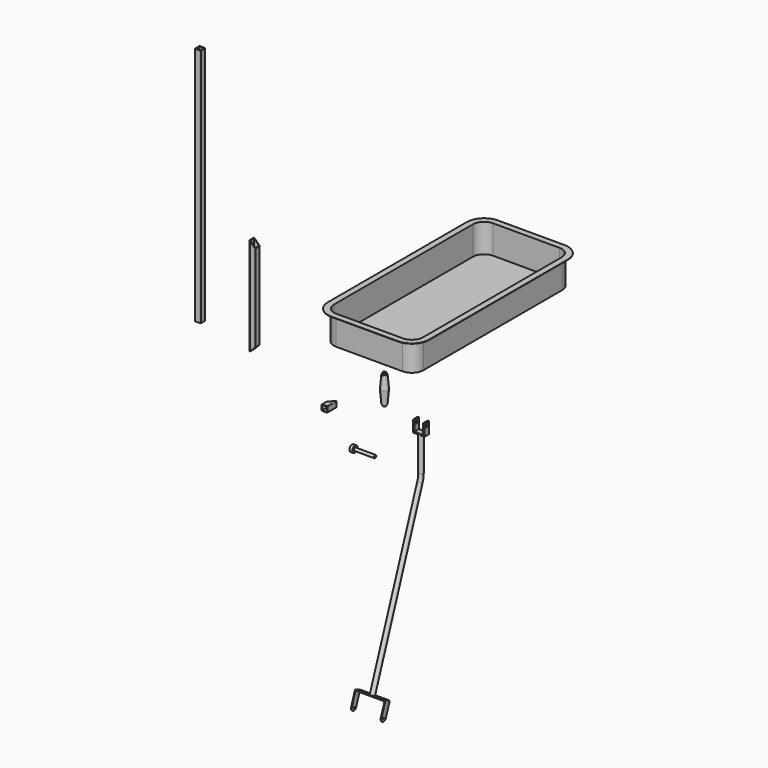
from build123d import *

# Parameters (mm, degrees)
F1_DEPTH  = 1054.1
F3_DEPTH  = 431.8
F5_DEPTH  = 50.8
F7_DEPTH  = 25.4
F9_DEPTH  = 25.4
F13_DEPTH = 127
F14_T     = -1.524
F16_DEPTH = 1.524
F18_DEPTH = 25.4
F19_R     = 9.525
F23_R     = 6.35
F24_DEPTH = 50.8
F25_W     = 127
F25_H     = 25.4
F25_R     = 9.525
F26_DEPTH = 3.175
F28_DEPTH = 25.4
F29_R     = 3.175
F30_DEPTH = 133.35
F31_R     = 12.69999


# Not quite as in the source:
# - a fillet or chamfer is up to 0.001 mm smaller than in the source, because OpenCascade refuses the exact size


with BuildPart() as f1:
    # F0 (on Top) → F1 (new body)
    with BuildSketch(Plane.XY):
        with BuildLine():
            ThreePointArc((-1008.6002467976, 278.8412709408), (-1007.9306928994, 277.224824839), (-1006.3142467976, 276.5552709408))
            Line((-1006.3142467976, 276.5552709408), (-985.4862467976, 276.5552709408))
            ThreePointArc((-985.4862467976, 276.5552709408), (-983.8698006958, 277.224824839), (-983.2002467976, 278.8412709408))
            Line((-983.2002467976, 278.8412709408), (-983.2002467976, 299.6692709408))
            ThreePointArc((-983.2002467976, 299.6692709408), (-983.8698006958, 301.2857170426), (-985.4862467976, 301.9552709408))
            Line((-985.4862467976, 301.9552709408), (-1006.3142467976, 301.9552709408))
            ThreePointArc((-1006.3142467976, 301.9552709408), (-1007.9306928994, 301.2857170426), (-1008.6002467976, 299.6692709408))
            Line((-1008.6002467976, 299.6692709408), (-1008.6002467976, 278.8412709408))
        make_face()
        with BuildLine():
            ThreePointArc((-1006.5682467976, 299.6692709408), (-1006.49385192, 299.8488760632), (-1006.3142467976, 299.9232709408))
            Line((-1006.3142467976, 299.9232709408), (-985.4862467976, 299.9232709408))
            ThreePointArc((-985.4862467976, 299.9232709408), (-985.3066416751, 299.8488760632), (-985.2322467976, 299.6692709408))
            Line((-985.2322467976, 299.6692709408), (-985.2322467976, 278.8412709408))
            ThreePointArc((-985.2322467976, 278.8412709408), (-985.3066416751, 278.6616658184), (-985.4862467976, 278.5872709408))
            Line((-985.4862467976, 278.5872709408), (-1006.3142467976, 278.5872709408))
            ThreePointArc((-1006.3142467976, 278.5872709408), (-1006.49385192, 278.6616658184), (-1006.5682467976, 278.8412709408))
            Line((-1006.5682467976, 278.8412709408), (-1006.5682467976, 299.6692709408))
        make_face(mode=Mode.SUBTRACT)
    extrude(amount=F1_DEPTH)


with BuildPart() as f3:
    # F2 (on Top) → F3 (new body)
    with BuildSketch(Plane.XY):
        with BuildLine():
            ThreePointArc((-720.8398963928, 218.5947193251), (-720.1703424946, 216.9782732233), (-718.5538963928, 216.3087193251))
            Line((-718.5538963928, 216.3087193251), (-697.7258963928, 216.3087193251))
            ThreePointArc((-697.7258963928, 216.3087193251), (-696.109450291, 216.9782732233), (-695.4398963928, 218.5947193251))
            Line((-695.4398963928, 218.5947193251), (-695.4398963928, 239.4227193251))
            ThreePointArc((-695.4398963928, 239.4227193251), (-696.109450291, 241.0391654269), (-697.7258963928, 241.7087193251))
            Line((-697.7258963928, 241.7087193251), (-718.5538963928, 241.7087193251))
            ThreePointArc((-718.5538963928, 241.7087193251), (-720.1703424946, 241.0391654269), (-720.8398963928, 239.4227193251))
            Line((-720.8398963928, 239.4227193251), (-720.8398963928, 218.5947193251))
        make_face()
        with BuildLine():
            ThreePointArc((-718.8078963928, 239.4227193251), (-718.7335015152, 239.6023244475), (-718.5538963928, 239.6767193251))
            Line((-718.5538963928, 239.6767193251), (-697.7258963928, 239.6767193251))
            ThreePointArc((-697.7258963928, 239.6767193251), (-697.5462912704, 239.6023244475), (-697.4718963928, 239.4227193251))
            Line((-697.4718963928, 239.4227193251), (-697.4718963928, 218.5947193251))
            ThreePointArc((-697.4718963928, 218.5947193251), (-697.5462912704, 218.4151142026), (-697.7258963928, 218.3407193251))
            Line((-697.7258963928, 218.3407193251), (-718.5538963928, 218.3407193251))
            ThreePointArc((-718.5538963928, 218.3407193251), (-718.7335015152, 218.4151142026), (-718.8078963928, 218.5947193251))
            Line((-718.8078963928, 218.5947193251), (-718.8078963928, 239.4227193251))
        make_face(mode=Mode.SUBTRACT)
    extrude(amount=F3_DEPTH)

    # F8 (on face) → F9 (cut, through all)
    with BuildSketch(Plane(origin=(0, 241.7087193251, 0), x_dir=(-1, 0, 0), z_dir=(0, 1, 0))):
        Polygon((695.4398963928, 431.8), (695.4398963928, 406.4), (697.7258963928, 408.686), (697.7258963928, 431.8), align=None)
        Polygon((697.7258963928, 431.8), (697.7258963928, 408.686), (718.5538963928, 429.514), (718.5538963928, 431.8), align=None)
        Polygon((718.5538963928, 431.8), (718.5538963928, 429.514), (720.8398963928, 431.8), align=None)
        Polygon((718.5538963928, 2.286), (697.7258963928, 23.114), (697.7258963928, 0), (718.5538963928, 0), align=None)
        Polygon((720.8398963928, 0), (718.5538963928, 2.286), (718.5538963928, 0), align=None)
        Polygon((697.7258963928, 0), (697.7258963928, 23.114), (695.4398963928, 25.4), (695.4398963928, 0), align=None)
    extrude(amount=-F9_DEPTH, mode=Mode.SUBTRACT)


with BuildPart() as f5:
    # F4 (on Front) → F5 (new body)
    with BuildSketch(Plane.XZ):
        with BuildLine():
            ThreePointArc((-190.3155680418, 55.463430141), (-189.6460141436, 53.8469840392), (-188.0295680418, 53.177430141))
            Line((-188.0295680418, 53.177430141), (-167.2015680418, 53.177430141))
            ThreePointArc((-167.2015680418, 53.177430141), (-165.58512194, 53.8469840392), (-164.9155680418, 55.463430141))
            Line((-164.9155680418, 55.463430141), (-164.9155680418, 76.291430141))
            ThreePointArc((-164.9155680418, 76.291430141), (-165.58512194, 77.9078762428), (-167.2015680418, 78.577430141))
            Line((-167.2015680418, 78.577430141), (-188.0295680418, 78.577430141))
            ThreePointArc((-188.0295680418, 78.577430141), (-189.6460141436, 77.9078762428), (-190.3155680418, 76.291430141))
            Line((-190.3155680418, 76.291430141), (-190.3155680418, 55.463430141))
        make_face()
        with BuildLine():
            ThreePointArc((-188.2835680418, 76.291430141), (-188.2091731642, 76.4710352634), (-188.0295680418, 76.545430141))
            Line((-188.0295680418, 76.545430141), (-167.2015680418, 76.545430141))
            ThreePointArc((-167.2015680418, 76.545430141), (-167.0219629194, 76.4710352634), (-166.9475680418, 76.291430141))
            Line((-166.9475680418, 76.291430141), (-166.9475680418, 55.463430141))
            ThreePointArc((-166.9475680418, 55.463430141), (-167.0219629194, 55.2838250186), (-167.2015680418, 55.209430141))
            Line((-167.2015680418, 55.209430141), (-188.0295680418, 55.209430141))
            ThreePointArc((-188.0295680418, 55.209430141), (-188.2091731642, 55.2838250186), (-188.2835680418, 55.463430141))
            Line((-188.2835680418, 55.463430141), (-188.2835680418, 76.291430141))
        make_face(mode=Mode.SUBTRACT)
    extrude(amount=F5_DEPTH)

    # F6 (on face) → F7 (cut, through all)
    with BuildSketch(Plane.XY.offset(78.577430141)):
        Polygon((-188.0295680418, 0), (-190.3155680418, 0), (-190.3155680418, -25.4), (-188.0295680418, -23.114), align=None)
        Polygon((-167.2015680418, 0), (-188.0295680418, 0), (-188.0295680418, -23.114), (-167.2015680418, -2.286), align=None)
        Polygon((-164.9155680418, 0), (-167.2015680418, 0), (-167.2015680418, -2.286), align=None)
    extrude(amount=-F7_DEPTH, mode=Mode.SUBTRACT)


with BuildPart() as f11:
    # F10 (on Top) → F11 (revolve)
    with BuildSketch(Plane.XY):
        Polygon((102.1386031211, -128.7457447313), (102.1386031211, -122.3957447313), (0.5386031211, -122.3957447313), (0.5386031211, -136.6832447313), (13.2386031211, -136.6832447313), (13.2386031211, -128.7457447313), align=None)
    revolve(axis=Axis((51.3386031211, -122.3957447313, 0), (-1, 0, 0)))


with BuildPart() as f13:
    # F12 (on Top) → F13 (new body)
    with BuildSketch(Plane.XY):
        with BuildLine():
            Line((-220.3151675584, 1294.6406504526), (-512.4151675584, 1294.6406504526))
            ThreePointArc((-512.4151675584, 1294.6406504526), (-548.3361920427, 1279.7616749369), (-563.2151675584, 1243.8406504526))
            Line((-563.2151675584, 1243.8406504526), (-563.2151675584, 481.8406504526))
            ThreePointArc((-563.2151675584, 481.8406504526), (-548.3361920427, 445.9196259683), (-512.4151675584, 431.0406504526))
            Line((-512.4151675584, 431.0406504526), (-220.3151675584, 431.0406504526))
            ThreePointArc((-220.3151675584, 431.0406504526), (-184.3941430741, 445.9196259683), (-169.5151675584, 481.8406504526))
            Line((-169.5151675584, 481.8406504526), (-169.5151675584, 1243.8406504526))
            ThreePointArc((-169.5151675584, 1243.8406504526), (-184.3941430741, 1279.7616749369), (-220.3151675584, 1294.6406504526))
        make_face()
    extrude(amount=F13_DEPTH)

    # F14
    f14_openings = [f13.faces().sort_by_distance(p)[0] for p in [
        (-366.365168, 862.84065, 127),
    ]]
    offset(amount=F14_T, openings=f14_openings)

    # F15 (on face) → F16 (join)
    with BuildSketch(Plane.XY.offset(127)):
        with BuildLine():
            Line((-220.3151675584, 1320.0406504526), (-512.4151675584, 1320.0406504526))
            ThreePointArc((-512.4151675584, 1320.0406504526), (-566.2967042848, 1297.722187179), (-588.6151675584, 1243.8406504526))
            Line((-588.6151675584, 1243.8406504526), (-588.6151675584, 481.8406504526))
            ThreePointArc((-588.6151675584, 481.8406504526), (-566.2967042848, 427.9591137262), (-512.4151675584, 405.6406504526))
            Line((-512.4151675584, 405.6406504526), (-220.3151675584, 405.6406504526))
            ThreePointArc((-220.3151675584, 405.6406504526), (-166.433630832, 427.9591137262), (-144.1151675584, 481.8406504526))
            Line((-144.1151675584, 481.8406504526), (-144.1151675584, 1243.8406504526))
            ThreePointArc((-144.1151675584, 1243.8406504526), (-166.433630832, 1297.722187179), (-220.3151675584, 1320.0406504526))
        make_face()
        with BuildLine():
            Line((-563.2151675584, 481.8406504526), (-563.2151675584, 1243.8406504526))
            ThreePointArc((-563.2151675584, 1243.8406504526), (-548.3361920427, 1279.7616749369), (-512.4151675584, 1294.6406504526))
            Line((-512.4151675584, 1294.6406504526), (-220.3151675584, 1294.6406504526))
            ThreePointArc((-220.3151675584, 1294.6406504526), (-184.3941430741, 1279.7616749369), (-169.5151675584, 1243.8406504526))
            Line((-169.5151675584, 1243.8406504526), (-169.5151675584, 481.8406504526))
            ThreePointArc((-169.5151675584, 481.8406504526), (-184.3941430741, 445.9196259683), (-220.3151675584, 431.0406504526))
            Line((-220.3151675584, 431.0406504526), (-512.4151675584, 431.0406504526))
            ThreePointArc((-512.4151675584, 431.0406504526), (-548.3361920427, 445.9196259683), (-563.2151675584, 481.8406504526))
        make_face(mode=Mode.SUBTRACT)
    extrude(amount=-F16_DEPTH)


with BuildPart() as f18:
    # F17 (on Front) → F18 (new body)
    with BuildSketch(Plane.XZ):
        Polygon((196.633880581, 133.0408798925), (190.283880581, 133.0408798925), (190.283880581, 82.2408798925), (241.083880581, 82.2408798925), (241.083880581, 133.0408798925), (234.733880581, 133.0408798925), (234.733880581, 87.9394591683), (196.633880581, 87.9394591683), align=None)
    extrude(amount=F18_DEPTH)

    # F22: sweep along a path in F21
    with BuildLine(Plane.YZ.offset(215.683880581)) as f22_path:
        Line((-12.7, 82.2408798925), (-12.7, -70.1591201075))
        ThreePointArc((-12.7, -70.1591201075), (-14.243532294, -87.8017749585), (-18.8272297282, -104.9083666694))
        Line((-18.8272297282, -104.9083666694), (-279.4465789423, -820.9541437083))
    # F19 (on face) → F22 (sweep)
    with BuildSketch(Plane(origin=(0, 0, 82.2408798925), x_dir=(1, 0, 0), z_dir=(0, 0, -1))):
        with Locations((215.683880581, 12.7)):
            Circle(F19_R)
    sweep(path=f22_path.line)

    # F23 (on face) → F24 (cut, through all)
    with BuildSketch(Plane.YZ.offset(241.083880581)):
        with Locations((-12.7, 120.3408798925)):
            Circle(F23_R)
    extrude(amount=-F24_DEPTH, mode=Mode.SUBTRACT)

    # F25 (on face) → F26 (join)
    with BuildSketch(Plane(origin=(0, -296.5386158457, -814.7331510325), x_dir=(1, 0, 0), z_dir=(0, -0.3420201433, -0.9396926208))):
        with Locations((215.683880581, -18.188965759)):
            Rectangle(F25_W, F25_H)
        with Locations((215.683880581, -18.188965759)):
            Circle(F25_R, mode=Mode.SUBTRACT)
        with Locations((215.683880581, -18.188965759)):
            Circle(F25_R)
    extrude(amount=F26_DEPTH)

    # F27 (on face) → F28 (join, through all)
    with BuildSketch(Plane(origin=(0, 5.1579406194, -1.8773368556), x_dir=(1, 0, 0), z_dir=(0, -0.9396926208, 0.3420201433))):
        Polygon((152.183880581, -870.195909828), (152.183880581, -867.020909828), (149.008880581, -867.020909828), (149.008880581, -943.220909828), (152.183880581, -943.220909828), align=None)
        Polygon((282.358880581, -867.020909828), (279.183880581, -867.020909828), (279.183880581, -870.195909828), (279.183880581, -943.220909828), (282.358880581, -943.220909828), align=None)
    extrude(amount=-F28_DEPTH)

    # F29 (on face) → F30 (cut, through all)
    with BuildSketch(Plane.YZ.offset(282.358880581)):
        with Locations((-301.1648580435, -880.6246251282)):
            Circle(F29_R)
    extrude(amount=-F30_DEPTH, mode=Mode.SUBTRACT)

    # F31 (radius 12.7 in the source; OpenCascade refuses exactly that, so slightly less here)
    f31_edges = [f18.edges().sort_by_distance(p)[0] for p in [
        (280.771381, -293.574418, -896.902377),
        (280.771381, -317.44261, -888.215066),
        (150.596381, -293.574418, -896.902377),
        (150.596381, -317.44261, -888.215066),
    ]]
    fillet(f31_edges, radius=F31_R)


with BuildPart() as f33:
    # F32 (on Front) → F33 (revolve)
    with BuildSketch(Plane.XZ):
        Polygon((60.973200519, 193.168364866), (55.9732233985, 250.318364866), (52.7982233985, 250.318364866), (52.7982233985, 256.668364866), (45.1782233985, 256.668364866), (45.1782233985, 129.668364866), (52.7982233985, 129.668364866), (52.7982233985, 136.018364866), (55.9732233985, 136.018364866), align=None)
    revolve(axis=Axis((45.1782233985, 0, 193.168364866), (0, 0, 1)))


solid = Compound([f1.part, f3.part, f5.part, f11.part, f13.part, f18.part, f33.part])
